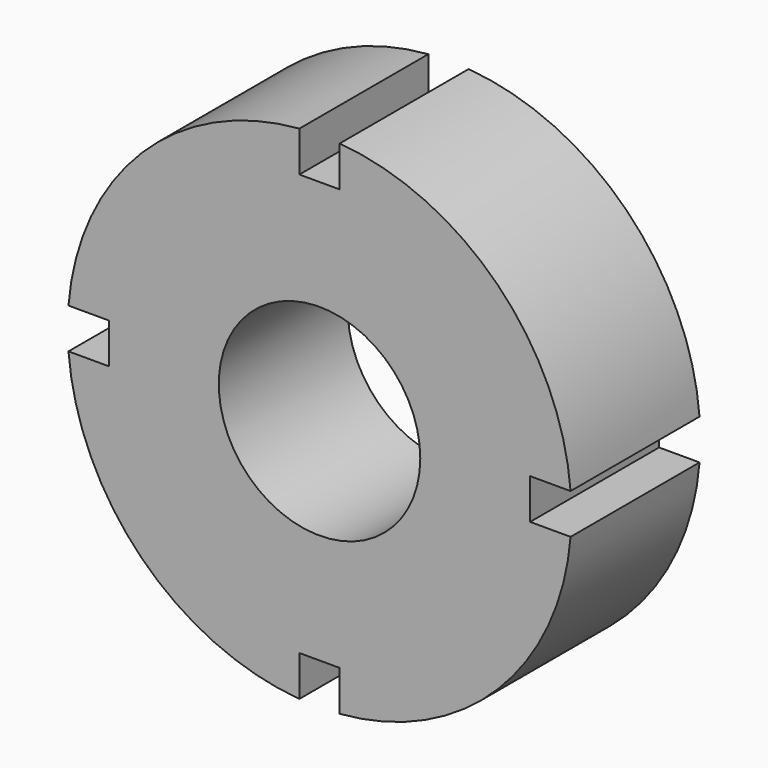
from build123d import *

# Parameters (mm, degrees)
F0_R            = 12.5
F0_R_2          = 5
F1_DEPTH        = 4
F3_DEPTH        = 25
F3_COPIES_COUNT = 4


# Not quite as in the source:
# - a pattern or mirror of a feature is missing from the dataset's text; its kind, count and spacing are read off the source's solid


with BuildPart() as f1:
    # F0 (on Front) → F1 (new body, symmetric)
    with BuildSketch(Plane.XZ):
        Circle(F0_R)
        Circle(F0_R_2, mode=Mode.SUBTRACT)
    extrude(amount=F1_DEPTH, both=True)

    # F2 (on face) → F3 (cut)
    with BuildSketch(Plane.XZ.offset(4)):
        with BuildLine():
            Line((10.4522724802, 1), (10.4522724802, -1))
            Line((10.4522724802, -1), (12.4599357944, -1))
            ThreePointArc((12.4599357944, -1), (12.4899799325, -0.5004011242), (12.5, 0))
            ThreePointArc((12.5, 0), (12.4899799325, 0.5004011242), (12.4599357944, 1))
            Line((12.4599357944, 1), (10.4522724802, 1))
        make_face()
    f3 = extrude(amount=-F3_DEPTH, mode=Mode.SUBTRACT)

    # F3_copies: F3 ×4 about axis
    f3_copies_axis = Axis((0, 0, 0), (0, 1, 0))
    for i in range(1, F3_COPIES_COUNT):
        add(f3.rotate(f3_copies_axis, i * 360 / F3_COPIES_COUNT), mode=Mode.SUBTRACT)


solid = f1.part
